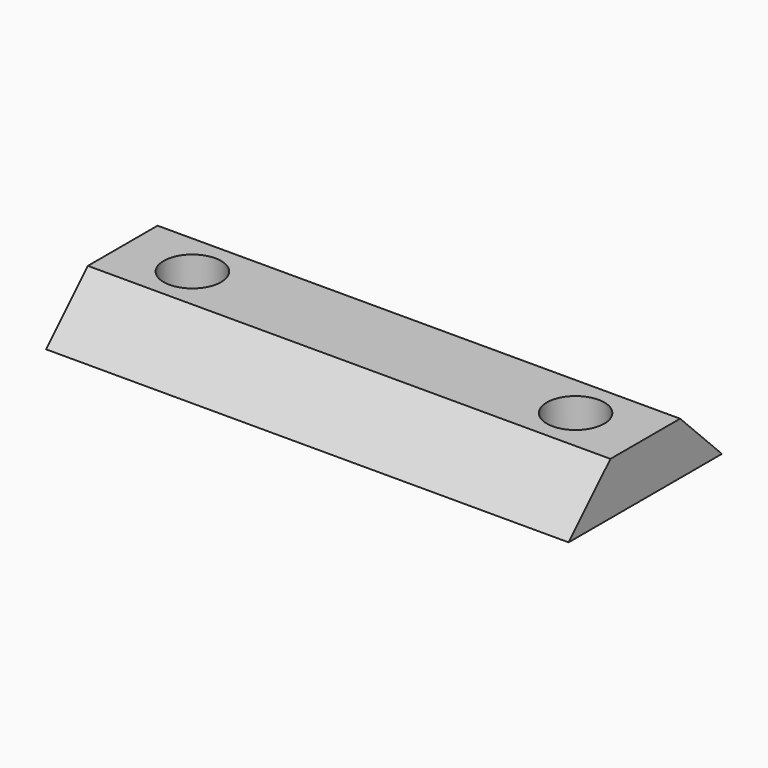
from build123d import *

# Parameters (mm, degrees)
F0_W     = 30
F0_H     = 11
F1_DEPTH = 3
F2_SIZE2 = 2.99999
F2_SIZE  = 2.99999
F3_D     = 3.3


# Not quite as in the source:
# - a fillet or chamfer is up to 0.001 mm smaller than in the source, because OpenCascade refuses the exact size


with BuildPart() as f1:
    # F0 (on Top) → F1 (new body)
    with BuildSketch(Plane.XY):
        with Locations((15, -5.5)):
            Rectangle(F0_W, F0_H)
    extrude(amount=F1_DEPTH)

    # F2 (size 3 and 3 in the source; OpenCascade refuses exactly that, so slightly less here)
    f2_edges = [f1.edges().sort_by_distance(p)[0] for p in [
        (15, -11, 3),
        (15, 0, 3),
    ]]
    chamfer(f2_edges, length=F2_SIZE, length2=F2_SIZE2)

    # F3 (through all)
    with Locations(Plane(origin=(0, 0, 0), x_dir=(1, 0, 0), z_dir=(0, 0, -1))):
        with Locations((4, 5.5), (26, 5.5)):
            Hole(F3_D / 2)


solid = f1.part
